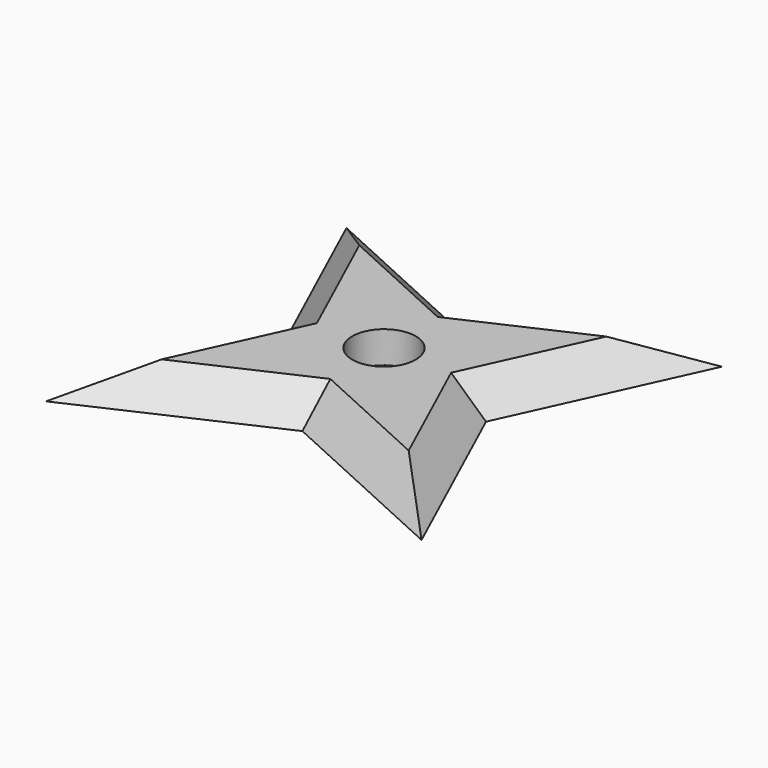
from build123d import *

# Parameters (mm, degrees)
F0_R     = 5.08
F1_DEPTH = 5.08
F2_SIZE  = 5.07999


# Not quite as in the source:
# - a fillet or chamfer is up to 0.001 mm smaller than in the source, because OpenCascade refuses the exact size


with BuildPart() as f1:
    # F0 (on Top) → F1 (new body)
    with BuildSketch(Plane.XY):
        with BuildLine():
            ThreePointArc((-16.3226491362, 0), (-11.5418558911, 11.5418558911), (0, 16.3226491362))
            Line((0, 16.3226491362), (-30.0371784096, 30.0371784096))
            Line((-30.0371784096, 30.0371784096), (-16.3226491362, 0))
        make_face()
        with BuildLine():
            ThreePointArc((0, 16.3226491362), (11.5418558911, 11.5418558911), (16.3226491362, 0))
            Line((16.3226491362, 0), (30.0371784096, 30.0371784096))
            Line((30.0371784096, 30.0371784096), (0, 16.3226491362))
        make_face()
        with BuildLine():
            Line((30.0371784096, -30.0371784096), (16.3226491362, 0))
            ThreePointArc((16.3226491362, 0), (11.5418558911, -11.5418558911), (0, -16.3226491362))
            Line((0, -16.3226491362), (30.0371784096, -30.0371784096))
        make_face()
        with BuildLine():
            Line((-30.0371784096, -30.0371784096), (0, -16.3226491362))
            ThreePointArc((0, -16.3226491362), (-11.5418558911, -11.5418558911), (-16.3226491362, 0))
            Line((-16.3226491362, 0), (-30.0371784096, -30.0371784096))
        make_face()
        with BuildLine():
            ThreePointArc((0, -16.3226491362), (11.5418558911, -11.5418558911), (16.3226491362, 0))
            ThreePointArc((16.3226491362, 0), (11.5418558911, 11.5418558911), (0, 16.3226491362))
            ThreePointArc((0, 16.3226491362), (-11.5418558911, 11.5418558911), (-16.3226491362, 0))
            ThreePointArc((-16.3226491362, 0), (-11.5418558911, -11.5418558911), (0, -16.3226491362))
        make_face()
        Circle(F0_R, mode=Mode.SUBTRACT)
    extrude(amount=F1_DEPTH)

    # F2 (size 5.08 in the source; OpenCascade refuses exactly that, so slightly less here)
    f2_edges = [f1.edges().sort_by_distance(p)[0] for p in [
        (-15.018589, -23.179914, 5.08),
        (-23.179914, -15.018589, 5.08),
        (15.018589, -23.179914, 5.08),
        (23.179914, -15.018589, 5.08),
        (23.179914, 15.018589, 5.08),
        (15.018589, 23.179914, 5.08),
        (-15.018589, 23.179914, 5.08),
        (-23.179914, 15.018589, 5.08),
    ]]
    chamfer(f2_edges, length=F2_SIZE)


solid = f1.part
